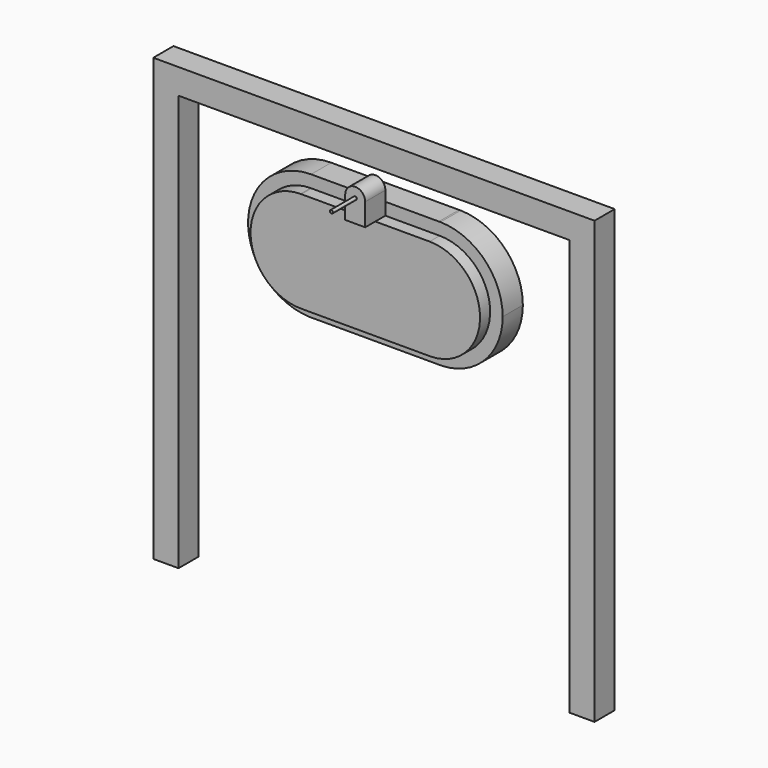
from build123d import *

# Parameters (mm, degrees)
F1_DEPTH = 25.4
F2_R     = 6.35
F3_DEPTH = 12.7
F2_R_2   = 1.5875
F4_DEPTH = 25.4
F5_DEPTH = 55.372
F6_DEPTH = 25.4
F8_DEPTH = 25.4


with BuildPart() as f1:
    # F0 (on Front) → F1 (new body)
    with BuildSketch(Plane.XZ):
        Polygon((220.7794714003, 444.5), (-223.7205285997, 444.5), (-223.7205285997, 0), (-198.3205285997, 0), (-198.3205285997, 419.1), (195.3794714003, 419.1), (195.3794714003, 0), (220.7794714003, 0), align=None)
    extrude(amount=-F1_DEPTH)


with BuildPart() as f3:
    # F2 (on face) → F3 (new body)
    with BuildSketch(Plane.XZ):
        with BuildLine():
            Line((-65.2600586708, 380.4436114409), (-64.3680339263, 380.4436249147))
            ThreePointArc((-64.3680339263, 380.4436249147), (-64.8140463281, 380.4455761588), (-65.2600586708, 380.4436114409))
        make_face()
        with BuildLine():
            Line((-10.0605708618, 380.4444452172), (-64.3680339263, 380.4436249147))
            Line((-64.3680339263, 380.4436249147), (-65.2600586708, 380.4436114409))
            ThreePointArc((-65.2600586708, 380.4436114409), (-115.6059339898, 328.7817476998), (-63.532459971, 278.8617253594))
            Line((-63.532459971, 278.8617253594), (63.532459971, 278.8617253594))
            Line((63.532459971, 278.8617253594), (66.0940980393, 278.8617253594))
            ThreePointArc((66.0940980393, 278.8617253594), (115.6092367076, 330.2864202149), (64.8125116822, 380.4455761588))
            Line((64.8125116822, 380.4455761588), (10.060519749, 380.4447491419))
            Line((10.060519749, 380.4447491419), (10.060519749, 330.9917804861))
            ThreePointArc((10.060519749, 330.9917804861), (10.0606420697, 330.963137726), (10.0606828434, 330.9344947338))
            ThreePointArc((10.0606828434, 330.9344947338), (10.0606420697, 330.9058517416), (10.060519749, 330.8772089815))
            ThreePointArc((10.060519749, 330.8772089815), (-0.0286543698, 320.8738526965), (-10.0606828434, 330.9345174891))
            Line((-10.0606828434, 330.9345174891), (-10.0605708618, 380.4444452172))
        make_face()
        with Locations((-65.0875, 330.2)):
            Circle(F2_R, mode=Mode.SUBTRACT)
        with Locations((65.0875, 330.2)):
            Circle(F2_R, mode=Mode.SUBTRACT)
        with BuildLine():
            Line((10.060519749, 380.4447491419), (-10.0605708618, 380.4444452172))
            Line((-10.0605708618, 380.4444452172), (-10.0606828434, 330.9345174891))
            ThreePointArc((-10.0606828434, 330.9345174891), (-0.0286316146, 340.9951368359), (10.060519749, 330.9917804861))
            Line((10.060519749, 330.9917804861), (10.060519749, 380.4447491419))
        make_face()
        with BuildLine():
            ThreePointArc((10.060519749, 330.9917804861), (-0.0286316146, 340.9951368359), (-10.0606828434, 330.9345174891))
            ThreePointArc((-10.0606828434, 330.9345174891), (-0.0286543698, 320.8738526965), (10.060519749, 330.8772089815))
            Line((10.060519749, 330.8772089815), (10.060519749, 330.9917804861))
        make_face()
        with BuildLine():
            Line((66.0940980393, 278.8617253594), (63.532459971, 278.8617253594))
            ThreePointArc((63.532459971, 278.8617253594), (64.8132790052, 278.8455761646), (66.0940980393, 278.8617253594))
        make_face()
        with BuildLine():
            ThreePointArc((10.0606828434, 330.9344947338), (10.0606420697, 330.963137726), (10.060519749, 330.9917804861))
            Line((10.060519749, 330.9917804861), (10.060519749, 330.8772089815))
            ThreePointArc((10.060519749, 330.8772089815), (10.0606420697, 330.9058517416), (10.0606828434, 330.9344947338))
        make_face()
        with Locations((-65.0875, 330.2)):
            Circle(F2_R)
        with Locations((65.0875, 330.2)):
            Circle(F2_R)
    extrude(amount=F3_DEPTH)

    # F2 (on face) → F4 (join)
    with BuildSketch(Plane.XZ):
        with BuildLine():
            Line((-10.060519749, 403.0427142477), (-10.0605708618, 380.4444452172))
            Line((-10.0605708618, 380.4444452172), (10.060519749, 380.4447491419))
            Line((10.060519749, 380.4447491419), (10.060519749, 403.0427142477))
            ThreePointArc((10.060519749, 403.0427142477), (0, 393.0393171566), (-10.060519749, 403.0427142477))
        make_face()
        with BuildLine():
            ThreePointArc((10.0606828434, 403.1), (-0.0286429922, 413.1606420697), (-10.060519749, 403.0427142477))
            ThreePointArc((-10.060519749, 403.0427142477), (0, 393.0393171566), (10.060519749, 403.0427142477))
            ThreePointArc((10.060519749, 403.0427142477), (10.0606420697, 403.0713570078), (10.0606828434, 403.1))
        make_face()
        with Locations((0, 403.1)):
            Circle(F2_R_2, mode=Mode.SUBTRACT)
    extrude(amount=F4_DEPTH)


with BuildPart() as f5:
    # F2 (on face) → F5 (new body)
    with BuildSketch(Plane.XZ):
        with Locations((0, 403.1)):
            Circle(F2_R_2)
    extrude(amount=F5_DEPTH)


with BuildPart() as f6:
    # F2 (on face) → F6 (new body)
    with BuildSketch(Plane.XZ):
        with Locations((65.0875, 330.2)):
            Circle(F2_R)
    extrude(amount=-F6_DEPTH)


with BuildPart() as f6b:
    # F2 (on face) → F6, piece 2 (new body)
    with BuildSketch(Plane.XZ):
        with Locations((-65.0875, 330.2)):
            Circle(F2_R)
    extrude(amount=-F6_DEPTH)


with BuildPart() as f8:
    # F7 (on face) → F8 (new body)
    with BuildSketch(Plane.XZ):
        with BuildLine():
            ThreePointArc((66.7321972552, 265.8258956615), (110.3404918101, 285.1031653263), (128.2404640913, 329.2946517467))
            ThreePointArc((128.2404640913, 329.2946517467), (109.916593326, 373.9193909323), (65.5202326779, 392.7898638572))
            Line((65.5202326779, 392.7898638572), (63.9653632353, 392.7899210088))
            ThreePointArc((63.9653632353, 392.7899210088), (1.24337931, 329.9031123291), (62.7487309274, 265.8258956615))
            Line((62.7487309274, 265.8258956615), (66.7321972552, 265.8258956615))
        make_face()
        with BuildLine():
            Line((63.9653632353, 392.7899210088), (65.5202326779, 392.7898638572))
            ThreePointArc((65.5202326779, 392.7898638572), (64.7427981316, 392.7946517039), (63.9653632353, 392.7899210088))
        make_face()
        with BuildLine():
            ThreePointArc((62.7487309274, 265.8258956615), (64.7404640913, 265.7946517467), (66.7321972552, 265.8258956615))
            Line((66.7321972552, 265.8258956615), (62.7487309274, 265.8258956615))
        make_face()
        with BuildLine():
            ThreePointArc((62.7487309274, 265.8258956615), (1.24337931, 329.9031123291), (63.9653632353, 392.7899210088))
            Line((63.9653632353, 392.7899210088), (-64.738130051, 392.7946517039))
            ThreePointArc((-64.738130051, 392.7946517039), (-19.8383582857, 374.1951071367), (-1.2404640913, 329.2946517467))
            ThreePointArc((-1.2404640913, 329.2946517467), (-19.1404363725, 285.1031653263), (-62.7487309274, 265.8258956615))
            Line((-62.7487309274, 265.8258956615), (62.7487309274, 265.8258956615))
        make_face()
        with BuildLine():
            ThreePointArc((-1.2404640913, 329.2946517467), (-19.8383582857, 374.1951071367), (-64.738130051, 392.7946517039))
            ThreePointArc((-64.738130051, 392.7946517039), (-128.2326343169, 330.2918077268), (-66.7321972552, 265.8258956615))
            Line((-66.7321972552, 265.8258956615), (-62.7487309274, 265.8258956615))
            ThreePointArc((-62.7487309274, 265.8258956615), (-19.1404363725, 285.1031653263), (-1.2404640913, 329.2946517467))
        make_face()
        with BuildLine():
            ThreePointArc((-66.7321972552, 265.8258956615), (-64.7404640913, 265.7946517467), (-62.7487309274, 265.8258956615))
            Line((-62.7487309274, 265.8258956615), (-66.7321972552, 265.8258956615))
        make_face()
    extrude(amount=-F8_DEPTH)


solid = Compound([f1.part, f3.part, f5.part, f6.part, f6b.part, f8.part])
